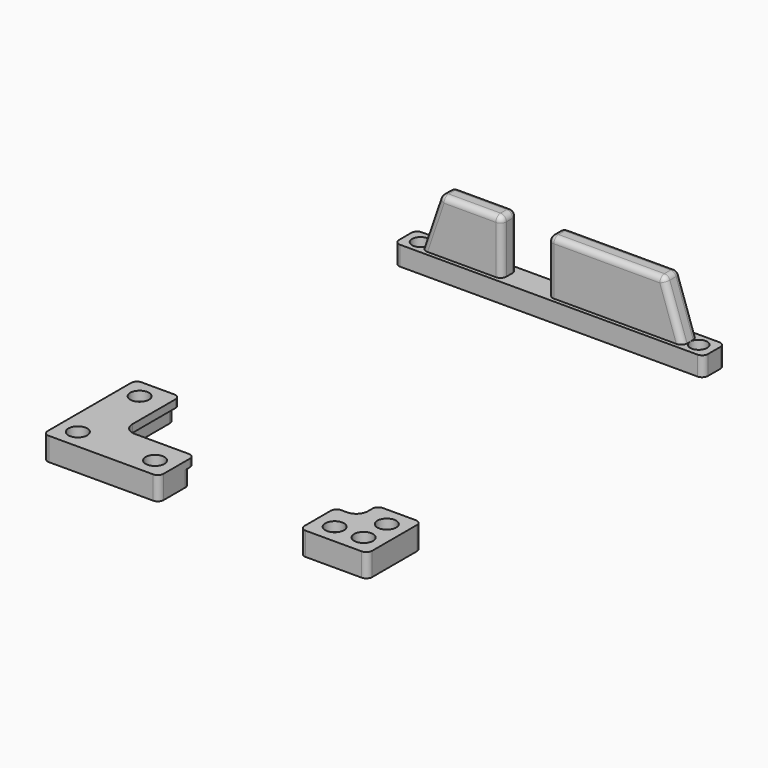
from build123d import *

# Parameters (mm, degrees)
F1_DEPTH         = 8
F4_DEPTH         = 4
F5_R             = 2.99999
F5_2_R           = 2.99999
F6_R             = 6
F6_2_R           = 6
F8_D             = 5.5
F8_DEPTH         = 40
F8_CBORE_D       = 9.75
F8_CBORE_DEPTH   = 5
F8_TIP           = 1.6523667023
F8_2_D           = 5.5
F8_2_DEPTH       = 40
F8_2_CBORE_D     = 9.75
F8_2_CBORE_DEPTH = 5
F8_2_TIP         = 1.6523667023
F0_W             = 160
F0_H             = 14
F9_DEPTH         = 10
F10_W            = 32
F10_H            = 10
F10_W_2          = 60
F11_DEPTH        = 28
F12_D            = 8.8
F12_DEPTH        = 15.75
F12_TIP          = 2.6437867237
F14_DEPTH        = 10
F15_R            = 3


# Not quite as in the source:
# - a fillet or chamfer is up to 0.001 mm smaller than in the source, because OpenCascade refuses the exact size


with BuildPart() as f1:
    # F0 (on Top) → F1 (new body)
    with BuildSketch(Plane.XY):
        Polygon((-24, -114), (-64, -114), (-64, -74), (-84, -74), (-84, -134), (-24, -134), align=None)
    extrude(amount=F1_DEPTH)

    # F3 (on face) → F4 (join)
    with BuildSketch(Plane.XY.offset(8)):
        Polygon((-61, -74), (-64, -74), (-64, -114), (-24, -114), (-24, -111), (-61, -111), align=None)
        Polygon((-64, -74), (-84, -74), (-84, -134), (-24, -134), (-24, -114), (-64, -114), align=None)
    extrude(amount=F4_DEPTH)

    # F5 (radius 3 in the source; OpenCascade refuses exactly that, so slightly less here)
    f5_edges = [f1.edges().sort_by_distance(p)[0] for p in [
        (-84, -134, 6),
        (-24, -134, 6),
        (-84, -74, 6),
        (-64, -74, 4),
        (-24, -114, 4),
        (-61, -74, 10),
        (-24, -111, 10),
    ]]
    fillet(f5_edges, radius=F5_R)

    # F6#2
    f6_2_edges = [f1.edges().sort_by_distance(p)[0] for p in [
        (-64, -114, 4),
        (-61, -111, 10),
    ]]
    fillet(f6_2_edges, radius=F6_2_R)

    # F8
    with Locations(Plane.XY.offset(12)):
        with Locations((-74, -124), (-74, -84), (-34, -124), (59, -124), (74, -124), (74, -109)):
            CounterBoreHole(F8_D / 2, F8_CBORE_D / 2, F8_CBORE_DEPTH, depth=F8_DEPTH)
            with Locations((0, 0, -(F8_DEPTH + F8_TIP / 2))):  # 118° drill point
                Cone(0, F8_D / 2, F8_TIP, mode=Mode.SUBTRACT)


with BuildPart() as f1b:
    # F0 (on Top) → F1, piece 2 (new body)
    with BuildSketch(Plane.XY):
        Polygon((64, -99), (64, -114), (49, -114), (49, -134), (84, -134), (84, -99), align=None)
    extrude(amount=F1_DEPTH)

    # F3 (on face) → F4, piece 2 (join)
    with BuildSketch(Plane.XY.offset(8)):
        Polygon((49, -111), (49, -134), (84, -134), (84, -99), (61, -99), (61, -111), align=None)
    extrude(amount=F4_DEPTH)

    # F5#2 (radius 3 in the source; OpenCascade refuses exactly that, so slightly less here)
    f5_2_edges = [f1b.edges().sort_by_distance(p)[0] for p in [
        (49, -134, 6),
        (84, -134, 6),
        (84, -99, 6),
        (49, -114, 4),
        (64, -99, 4),
        (49, -111, 10),
        (61, -99, 10),
    ]]
    fillet(f5_2_edges, radius=F5_2_R)

    # F6
    f6_edges = [f1b.edges().sort_by_distance(p)[0] for p in [
        (64, -114, 4),
        (61, -111, 10),
    ]]
    fillet(f6_edges, radius=F6_R)

    # F8#2
    with Locations(Plane.XY.offset(12)):
        with Locations((-74, -124), (-74, -84), (-34, -124), (59, -124), (74, -124), (74, -109)):
            CounterBoreHole(F8_2_D / 2, F8_2_CBORE_D / 2, F8_2_CBORE_DEPTH, depth=F8_2_DEPTH)
            with Locations((0, 0, -(F8_2_DEPTH + F8_2_TIP / 2))):  # 118° drill point
                Cone(0, F8_2_D / 2, F8_2_TIP, mode=Mode.SUBTRACT)


with BuildPart() as f9:
    # F0 (on Top) → F9 (new body)
    with BuildSketch(Plane.XY):
        with Locations((0, 95.388181746)):
            Rectangle(F0_W, F0_H)
    extrude(amount=F9_DEPTH)

    # F10 (on face) → F11 (join)
    with BuildSketch(Plane.XY.offset(10)):
        with Locations((-42, 95.388181746)):
            Rectangle(F10_W, F10_H)
        with Locations((28, 95.388181746)):
            Rectangle(F10_W_2, F10_H)
    extrude(amount=F11_DEPTH)

    # F12
    with Locations(Plane(origin=(0, 0, 0), x_dir=(1, 0, 0), z_dir=(0, 0, -1))):
        with Locations((-72, -95.388181746), (72, -95.388181746)):
            Hole(F12_D / 2, depth=F12_DEPTH)
            with Locations((0, 0, -(F12_DEPTH + F12_TIP / 2))):  # 118° drill point
                Cone(0, F12_D / 2, F12_TIP, mode=Mode.SUBTRACT)

    # F13 (on face) → F14 (join, through all)
    with BuildSketch(Plane.XZ.offset(-90.388181746)):
        Polygon((-58, 38), (-67.6, 10), (-58, 10), align=None)
        Polygon((58, 10), (67.6, 10), (58, 38), align=None)
    extrude(amount=-F14_DEPTH)

    # F15
    f15_edges = [f9.edges().sort_by_distance(p)[0] for p in [
        (-80, 88.388182, 5),
        (-80, 102.388182, 5),
        (80, 88.388182, 5),
        (80, 102.388182, 5),
        (62.8, 100.388182, 24),
        (62.8, 90.388182, 24),
        (-62.8, 100.388182, 24),
        (-62.8, 90.388182, 24),
        (-2, 100.388182, 24),
        (-2, 90.388182, 24),
        (-26, 90.388182, 24),
        (-26, 100.388182, 24),
        (-42, 100.388182, 38),
        (-42, 90.388182, 38),
        (28, 90.388182, 38),
        (28, 100.388182, 38),
        (-2, 95.388182, 38),
        (-26, 95.388182, 38),
        (-58, 95.388182, 38),
        (58, 95.388182, 38),
    ]]
    fillet(f15_edges, radius=F15_R)


solid = Compound([f1.part, f1b.part, f9.part])
